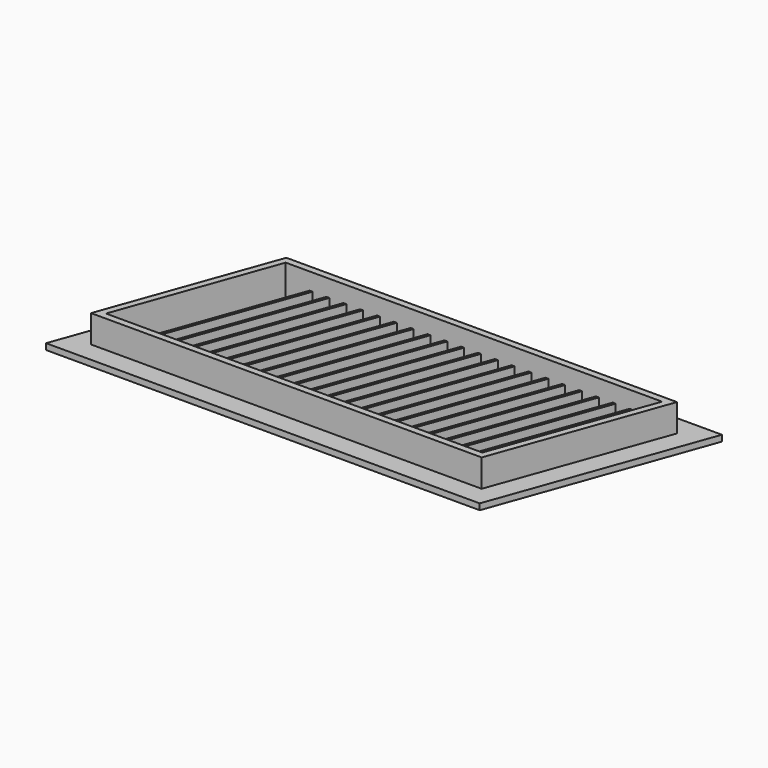
from build123d import *

# Parameters (mm, degrees)
F1_DEPTH      = 1.8
F2_DEPTH      = 5
F3_DEPTH      = 10
F4_T4_DEPTH   = 59.1767472924
F4_T10_DEPTH  = 59.1767472924
F4_T16_DEPTH  = 59.1767472924
F4_T22_DEPTH  = 59.1767472924
F4_T28_DEPTH  = 59.1767472924
F4_T34_DEPTH  = 59.1767472924
F4_T40_DEPTH  = 59.1767472924
F4_T46_DEPTH  = 59.1767472924
F4_T52_DEPTH  = 59.1767472924
F4_T58_DEPTH  = 59.1767472924
F4_T64_DEPTH  = 59.1767472924
F4_T70_DEPTH  = 59.1767472924
F4_T76_DEPTH  = 59.1767472924
F4_T82_DEPTH  = 59.1767472924
F4_T88_DEPTH  = 59.1767472924
F4_T94_DEPTH  = 59.1767472924
F4_T100_DEPTH = 59.1767472924
F4_T106_DEPTH = 59.1767472924
F4_T112_DEPTH = 59.1767472924
F4_T118_DEPTH = 59.1767472924
F4_T124_DEPTH = 59.1767472924
F4_T130_DEPTH = 59.1767472924
F4_T136_DEPTH = 59.1767472924
F4_T142_DEPTH = 59.1767472924
F4_T148_DEPTH = 59.1767472924
F4_T154_DEPTH = 59.1767472924
F4_T160_DEPTH = 59.1767472924
F4_T166_DEPTH = 59.1767472924
F4_T172_DEPTH = 59.1767472924
F4_T178_DEPTH = 59.1767472924
F4_T184_DEPTH = 59.1767472924
F4_T190_DEPTH = 59.1767472924
F4_T196_DEPTH = 59.1767472924
F4_T202_DEPTH = 59.1767472924
F4_T208_DEPTH = 59.1767472924
F4_T214_DEPTH = 59.1767472924
F4_T220_DEPTH = 59.1767472924
F4_T226_DEPTH = 59.1767472924
F4_T232_DEPTH = 59.1767472924
F4_T238_DEPTH = 59.1767472924
F4_T244_DEPTH = 59.1767472924
F4_T250_DEPTH = 59.1767472924
F4_T256_DEPTH = 59.1767472924


# Not quite as in the source:
# - a fillet or chamfer that OpenCascade refuses, or shapes differently, is made with other operations: its cross-section is extruded or revolved along the edge and cut away or added
# - a feature names something its author has since deleted; it is built from what else it names


with BuildPart() as f1:
    # F0 (on Top) → F1 (new body)
    with BuildSketch(Plane.XY):
        Polygon((4.2169585227, -6), (26.5369585227, 56), (-102.2169585227, 56), (-124.5369585227, -6), align=None)
        Polygon((-98, 0), (-116, 0), (-98, 50), (18, 50), (0, 0), align=None, mode=Mode.SUBTRACT)
    extrude(amount=F1_DEPTH)

    # F0 (on Top) → F2 (join)
    with BuildSketch(Plane.XY):
        Polygon((-98, 50), (-116, 0), (-98, 0), (0, 0), (18, 50), align=None)
        Polygon((13.4056528409, 48), (15.1543471591, 48), (-1.4056528409, 2), (-3.1543471591, 2), (-5.1543471591, 2), (-8.1543471591, 2), (-10.1543471591, 2), (-13.1543471591, 2), (-15.1543471591, 2), (-18.1543471591, 2), (-20.1543471591, 2), (-23.1543471591, 2), (-25.1543471591, 2), (-28.1543471591, 2), (-30.1543471591, 2), (-33.1543471591, 2), (-35.1543471591, 2), (-38.1543471591, 2), (-40.1543471591, 2), (-43.1543471591, 2), (-45.1543471591, 2), (-48.1543471591, 2), (-50.1543471591, 2), (-53.1543471591, 2), (-55.1543471591, 2), (-58.1543471591, 2), (-60.1543471591, 2), (-63.1543471591, 2), (-65.1543471591, 2), (-68.1543471591, 2), (-70.1543471591, 2), (-73.1543471591, 2), (-75.1543471591, 2), (-78.1543471591, 2), (-80.1543471591, 2), (-83.1543471591, 2), (-85.1543471591, 2), (-88.1543471591, 2), (-90.1543471591, 2), (-93.1543471591, 2), (-95.1543471591, 2), (-98.1543471591, 2), (-100.1543471591, 2), (-103.1543471591, 2), (-105.1543471591, 2), (-108.1543471591, 2), (-113.1543471591, 2), (-96.5943471591, 48), (-91.5943471591, 48), (-88.5943471591, 48), (-86.5943471591, 48), (-83.5943471591, 48), (-81.5943471591, 48), (-78.5943471591, 48), (-76.5943471591, 48), (-73.5943471591, 48), (-71.5943471591, 48), (-68.5943471591, 48), (-66.5943471591, 48), (-63.5943471591, 48), (-61.5943471591, 48), (-58.5943471591, 48), (-56.5943471591, 48), (-53.5943471591, 48), (-51.5943471591, 48), (-48.5943471591, 48), (-46.5943471591, 48), (-43.5943471591, 48), (-41.5943471591, 48), (-38.5943471591, 48), (-36.5943471591, 48), (-33.5943471591, 48), (-31.5943471591, 48), (-28.5943471591, 48), (-26.5943471591, 48), (-23.5943471591, 48), (-21.5943471591, 48), (-18.5943471591, 48), (-16.5943471591, 48), (-13.5943471591, 48), (-11.5943471591, 48), (-8.5943471591, 48), (-6.5943471591, 48), (-3.5943471591, 48), (-1.5943471591, 48), (1.4056528409, 48), (3.4056528409, 48), (6.4056528409, 48), (8.4056528409, 48), (11.4056528409, 48), align=None, mode=Mode.SUBTRACT)
        Polygon((-105.1543471591, 2), (-88.5943471591, 48), (-91.5943471591, 48), (-108.1543471591, 2), align=None)
        Polygon((-100.1543471591, 2), (-83.5943471591, 48), (-86.5943471591, 48), (-103.1543471591, 2), align=None)
        Polygon((-95.1543471591, 2), (-78.5943471591, 48), (-81.5943471591, 48), (-98.1543471591, 2), align=None)
        Polygon((-90.1543471591, 2), (-73.5943471591, 48), (-76.5943471591, 48), (-93.1543471591, 2), align=None)
        Polygon((-85.1543471591, 2), (-68.5943471591, 48), (-71.5943471591, 48), (-88.1543471591, 2), align=None)
        Polygon((-80.1543471591, 2), (-63.5943471591, 48), (-66.5943471591, 48), (-83.1543471591, 2), align=None)
        Polygon((-75.1543471591, 2), (-58.5943471591, 48), (-61.5943471591, 48), (-78.1543471591, 2), align=None)
        Polygon((-70.1543471591, 2), (-53.5943471591, 48), (-56.5943471591, 48), (-73.1543471591, 2), align=None)
        Polygon((-65.1543471591, 2), (-48.5943471591, 48), (-51.5943471591, 48), (-68.1543471591, 2), align=None)
        Polygon((-60.1543471591, 2), (-43.5943471591, 48), (-46.5943471591, 48), (-63.1543471591, 2), align=None)
        Polygon((-55.1543471591, 2), (-38.5943471591, 48), (-41.5943471591, 48), (-58.1543471591, 2), align=None)
        Polygon((-50.1543471591, 2), (-33.5943471591, 48), (-36.5943471591, 48), (-53.1543471591, 2), align=None)
        Polygon((-45.1543471591, 2), (-28.5943471591, 48), (-31.5943471591, 48), (-48.1543471591, 2), align=None)
        Polygon((-40.1543471591, 2), (-23.5943471591, 48), (-26.5943471591, 48), (-43.1543471591, 2), align=None)
        Polygon((-35.1543471591, 2), (-18.5943471591, 48), (-21.5943471591, 48), (-38.1543471591, 2), align=None)
        Polygon((-30.1543471591, 2), (-13.5943471591, 48), (-16.5943471591, 48), (-33.1543471591, 2), align=None)
        Polygon((-25.1543471591, 2), (-8.5943471591, 48), (-11.5943471591, 48), (-28.1543471591, 2), align=None)
        Polygon((-20.1543471591, 2), (-3.5943471591, 48), (-6.5943471591, 48), (-23.1543471591, 2), align=None)
        Polygon((-15.1543471591, 2), (1.4056528409, 48), (-1.5943471591, 48), (-18.1543471591, 2), align=None)
        Polygon((-10.1543471591, 2), (6.4056528409, 48), (3.4056528409, 48), (-13.1543471591, 2), align=None)
        Polygon((-5.1543471591, 2), (11.4056528409, 48), (8.4056528409, 48), (-8.1543471591, 2), align=None)
        Polygon((-1.4056528409, 2), (15.1543471591, 48), (13.4056528409, 48), (-3.1543471591, 2), align=None)
    extrude(amount=F2_DEPTH)

    # F0 (on Top) → F3 (join)
    with BuildSketch(Plane.XY):
        Polygon((-98, 50), (-116, 0), (-98, 0), (0, 0), (18, 50), align=None)
        Polygon((13.4056528409, 48), (15.1543471591, 48), (-1.4056528409, 2), (-3.1543471591, 2), (-5.1543471591, 2), (-8.1543471591, 2), (-10.1543471591, 2), (-13.1543471591, 2), (-15.1543471591, 2), (-18.1543471591, 2), (-20.1543471591, 2), (-23.1543471591, 2), (-25.1543471591, 2), (-28.1543471591, 2), (-30.1543471591, 2), (-33.1543471591, 2), (-35.1543471591, 2), (-38.1543471591, 2), (-40.1543471591, 2), (-43.1543471591, 2), (-45.1543471591, 2), (-48.1543471591, 2), (-50.1543471591, 2), (-53.1543471591, 2), (-55.1543471591, 2), (-58.1543471591, 2), (-60.1543471591, 2), (-63.1543471591, 2), (-65.1543471591, 2), (-68.1543471591, 2), (-70.1543471591, 2), (-73.1543471591, 2), (-75.1543471591, 2), (-78.1543471591, 2), (-80.1543471591, 2), (-83.1543471591, 2), (-85.1543471591, 2), (-88.1543471591, 2), (-90.1543471591, 2), (-93.1543471591, 2), (-95.1543471591, 2), (-98.1543471591, 2), (-100.1543471591, 2), (-103.1543471591, 2), (-105.1543471591, 2), (-108.1543471591, 2), (-113.1543471591, 2), (-96.5943471591, 48), (-91.5943471591, 48), (-88.5943471591, 48), (-86.5943471591, 48), (-83.5943471591, 48), (-81.5943471591, 48), (-78.5943471591, 48), (-76.5943471591, 48), (-73.5943471591, 48), (-71.5943471591, 48), (-68.5943471591, 48), (-66.5943471591, 48), (-63.5943471591, 48), (-61.5943471591, 48), (-58.5943471591, 48), (-56.5943471591, 48), (-53.5943471591, 48), (-51.5943471591, 48), (-48.5943471591, 48), (-46.5943471591, 48), (-43.5943471591, 48), (-41.5943471591, 48), (-38.5943471591, 48), (-36.5943471591, 48), (-33.5943471591, 48), (-31.5943471591, 48), (-28.5943471591, 48), (-26.5943471591, 48), (-23.5943471591, 48), (-21.5943471591, 48), (-18.5943471591, 48), (-16.5943471591, 48), (-13.5943471591, 48), (-11.5943471591, 48), (-8.5943471591, 48), (-6.5943471591, 48), (-3.5943471591, 48), (-1.5943471591, 48), (1.4056528409, 48), (3.4056528409, 48), (6.4056528409, 48), (8.4056528409, 48), (11.4056528409, 48), align=None, mode=Mode.SUBTRACT)
    extrude(amount=F3_DEPTH)

    # F4: chamfer of 2 on 43 edges, made by hand


with BuildPart() as f4_tool2:
    # F4_s3 → F4_t4 (new body)
    with BuildSketch(Plane(origin=(-8.0063254971, -22.2397930476, 0), x_dir=(0, 0, 1), z_dir=(0.3387194683, 0.9408874119, 0))):
        Polygon((2, -57.2759069477), (0, -59.2759069477), (0, -57.2759069477), align=None)
    extrude(amount=F4_T4_DEPTH)

    split(bisect_by=Plane.XZ.offset(-2), keep=Keep.BOTTOM)

    split(bisect_by=Plane.XZ.offset(-48), keep=Keep.TOP)


with BuildPart() as f1_1:
    add(f1.part)

    # F4_t1: cut F4_tool2
    add(f4_tool2.part, mode=Mode.SUBTRACT)


with BuildPart() as f4_tool8:
    # F4_s9 → F4_t10 (new body)
    with BuildSketch(Plane(origin=(-8.5799798881, -23.8332774668, 0), x_dir=(0, 0, 1), z_dir=(0.3387194683, 0.9408874119, 0))):
        Polygon((2, -61.9803440071), (0, -63.9803440071), (0, -61.9803440071), align=None)
    extrude(amount=F4_T10_DEPTH)

    split(bisect_by=Plane.XZ.offset(-2), keep=Keep.BOTTOM)

    split(bisect_by=Plane.XZ.offset(-48), keep=Keep.TOP)


with BuildPart() as f1_2:
    add(f1_1.part)

    # F4_t7: cut F4_tool8
    add(f4_tool8.part, mode=Mode.SUBTRACT)


with BuildPart() as f4_tool14:
    # F4_s15 → F4_t16 (new body)
    with BuildSketch(Plane(origin=(-9.153634279, -25.4267618861, 0), x_dir=(0, 0, 1), z_dir=(0.3387194683, 0.9408874119, 0))):
        Polygon((2, -66.6847810664), (0, -68.6847810664), (0, -66.6847810664), align=None)
    extrude(amount=F4_T16_DEPTH)

    split(bisect_by=Plane.XZ.offset(-2), keep=Keep.BOTTOM)

    split(bisect_by=Plane.XZ.offset(-48), keep=Keep.TOP)


with BuildPart() as f1_3:
    add(f1_2.part)

    # F4_t13: cut F4_tool14
    add(f4_tool14.part, mode=Mode.SUBTRACT)


with BuildPart() as f4_tool20:
    # F4_s21 → F4_t22 (new body)
    with BuildSketch(Plane(origin=(-9.7272886699, -27.0202463054, 0), x_dir=(0, 0, 1), z_dir=(0.3387194683, 0.9408874119, 0))):
        Polygon((2, -71.3892181258), (0, -73.3892181258), (0, -71.3892181258), align=None)
    extrude(amount=F4_T22_DEPTH)

    split(bisect_by=Plane.XZ.offset(-2), keep=Keep.BOTTOM)

    split(bisect_by=Plane.XZ.offset(-48), keep=Keep.TOP)


with BuildPart() as f1_4:
    add(f1_3.part)

    # F4_t19: cut F4_tool20
    add(f4_tool20.part, mode=Mode.SUBTRACT)


with BuildPart() as f4_tool26:
    # F4_s27 → F4_t28 (new body)
    with BuildSketch(Plane(origin=(-10.3009430609, -28.6137307246, 0), x_dir=(0, 0, 1), z_dir=(0.3387194683, 0.9408874119, 0))):
        Polygon((2, -76.0936551851), (0, -78.0936551851), (0, -76.0936551851), align=None)
    extrude(amount=F4_T28_DEPTH)

    split(bisect_by=Plane.XZ.offset(-2), keep=Keep.BOTTOM)

    split(bisect_by=Plane.XZ.offset(-48), keep=Keep.TOP)


with BuildPart() as f1_5:
    add(f1_4.part)

    # F4_t25: cut F4_tool26
    add(f4_tool26.part, mode=Mode.SUBTRACT)


with BuildPart() as f4_tool32:
    # F4_s33 → F4_t34 (new body)
    with BuildSketch(Plane(origin=(-10.8745974518, -30.2072151439, 0), x_dir=(0, 0, 1), z_dir=(0.3387194683, 0.9408874119, 0))):
        Polygon((2, -80.7980922444), (0, -82.7980922444), (0, -80.7980922444), align=None)
    extrude(amount=F4_T34_DEPTH)

    split(bisect_by=Plane.XZ.offset(-2), keep=Keep.BOTTOM)

    split(bisect_by=Plane.XZ.offset(-48), keep=Keep.TOP)


with BuildPart() as f1_6:
    add(f1_5.part)

    # F4_t31: cut F4_tool32
    add(f4_tool32.part, mode=Mode.SUBTRACT)


with BuildPart() as f4_tool38:
    # F4_s39 → F4_t40 (new body)
    with BuildSketch(Plane(origin=(-11.4482518427, -31.8006995631, 0), x_dir=(0, 0, 1), z_dir=(0.3387194683, 0.9408874119, 0))):
        Polygon((2, -85.5025293038), (0, -87.5025293038), (0, -85.5025293038), align=None)
    extrude(amount=F4_T40_DEPTH)

    split(bisect_by=Plane.XZ.offset(-2), keep=Keep.BOTTOM)

    split(bisect_by=Plane.XZ.offset(-48), keep=Keep.TOP)


with BuildPart() as f1_7:
    add(f1_6.part)

    # F4_t37: cut F4_tool38
    add(f4_tool38.part, mode=Mode.SUBTRACT)


with BuildPart() as f4_tool44:
    # F4_s45 → F4_t46 (new body)
    with BuildSketch(Plane(origin=(-12.0219062337, -33.3941839824, 0), x_dir=(0, 0, 1), z_dir=(0.3387194683, 0.9408874119, 0))):
        Polygon((2, -90.2069663631), (0, -92.2069663631), (0, -90.2069663631), align=None)
    extrude(amount=F4_T46_DEPTH)

    split(bisect_by=Plane.XZ.offset(-2), keep=Keep.BOTTOM)

    split(bisect_by=Plane.XZ.offset(-48), keep=Keep.TOP)


with BuildPart() as f1_8:
    add(f1_7.part)

    # F4_t43: cut F4_tool44
    add(f4_tool44.part, mode=Mode.SUBTRACT)


with BuildPart() as f4_tool50:
    # F4_s51 → F4_t52 (new body)
    with BuildSketch(Plane(origin=(-12.5955606246, -34.9876684017, 0), x_dir=(0, 0, 1), z_dir=(0.3387194683, 0.9408874119, 0))):
        Polygon((2, -94.9114034225), (0, -96.9114034225), (0, -94.9114034225), align=None)
    extrude(amount=F4_T52_DEPTH)

    split(bisect_by=Plane.XZ.offset(-2), keep=Keep.BOTTOM)

    split(bisect_by=Plane.XZ.offset(-48), keep=Keep.TOP)


with BuildPart() as f1_9:
    add(f1_8.part)

    # F4_t49: cut F4_tool50
    add(f4_tool50.part, mode=Mode.SUBTRACT)


with BuildPart() as f4_tool56:
    # F4_s57 → F4_t58 (new body)
    with BuildSketch(Plane(origin=(-13.1692150155, -36.5811528209, 0), x_dir=(0, 0, 1), z_dir=(0.3387194683, 0.9408874119, 0))):
        Polygon((2, -99.6158404818), (0, -101.6158404818), (0, -99.6158404818), align=None)
    extrude(amount=F4_T58_DEPTH)

    split(bisect_by=Plane.XZ.offset(-2), keep=Keep.BOTTOM)

    split(bisect_by=Plane.XZ.offset(-48), keep=Keep.TOP)


with BuildPart() as f1_10:
    add(f1_9.part)

    # F4_t55: cut F4_tool56
    add(f4_tool56.part, mode=Mode.SUBTRACT)


with BuildPart() as f4_tool62:
    # F4_s63 → F4_t64 (new body)
    with BuildSketch(Plane(origin=(11.6937982453, 32.4827729037, 0), x_dir=(0, 0, 1), z_dir=(-0.3387194683, -0.9408874119, 0))):
        Polygon((5, 58.0985691833), (3, 60.0985691833), (5, 60.0985691833), align=None)
    extrude(amount=F4_T64_DEPTH)

    split(bisect_by=Plane.XZ.offset(-2), keep=Keep.BOTTOM)

    split(bisect_by=Plane.XZ.offset(-48), keep=Keep.TOP)


with BuildPart() as f1_11:
    add(f1_10.part)

    # F4_t61: cut F4_tool62
    add(f4_tool62.part, mode=Mode.SUBTRACT)


with BuildPart() as f4_tool68:
    # F4_s69 → F4_t70 (new body)
    with BuildSketch(Plane(origin=(11.1201438544, 30.8892884844, 0), x_dir=(0, 0, 1), z_dir=(-0.3387194683, -0.9408874119, 0))):
        Polygon((5, 62.8030062427), (3, 64.8030062427), (5, 64.8030062427), align=None)
    extrude(amount=F4_T70_DEPTH)

    split(bisect_by=Plane.XZ.offset(-2), keep=Keep.BOTTOM)

    split(bisect_by=Plane.XZ.offset(-48), keep=Keep.TOP)


with BuildPart() as f1_12:
    add(f1_11.part)

    # F4_t67: cut F4_tool68
    add(f4_tool68.part, mode=Mode.SUBTRACT)


with BuildPart() as f4_tool74:
    # F4_s75 → F4_t76 (new body)
    with BuildSketch(Plane(origin=(10.5464894634, 29.2958040651, 0), x_dir=(0, 0, 1), z_dir=(-0.3387194683, -0.9408874119, 0))):
        Polygon((5, 67.507443302), (3, 69.507443302), (5, 69.507443302), align=None)
    extrude(amount=F4_T76_DEPTH)

    split(bisect_by=Plane.XZ.offset(-2), keep=Keep.BOTTOM)

    split(bisect_by=Plane.XZ.offset(-48), keep=Keep.TOP)


with BuildPart() as f1_13:
    add(f1_12.part)

    # F4_t73: cut F4_tool74
    add(f4_tool74.part, mode=Mode.SUBTRACT)


with BuildPart() as f4_tool80:
    # F4_s81 → F4_t82 (new body)
    with BuildSketch(Plane(origin=(9.9728350725, 27.7023196459, 0), x_dir=(0, 0, 1), z_dir=(-0.3387194683, -0.9408874119, 0))):
        Polygon((5, 72.2118803614), (3, 74.2118803614), (5, 74.2118803614), align=None)
    extrude(amount=F4_T82_DEPTH)

    split(bisect_by=Plane.XZ.offset(-2), keep=Keep.BOTTOM)

    split(bisect_by=Plane.XZ.offset(-48), keep=Keep.TOP)


with BuildPart() as f1_14:
    add(f1_13.part)

    # F4_t79: cut F4_tool80
    add(f4_tool80.part, mode=Mode.SUBTRACT)


with BuildPart() as f4_tool86:
    # F4_s87 → F4_t88 (new body)
    with BuildSketch(Plane(origin=(9.3991806816, 26.1088352266, 0), x_dir=(0, 0, 1), z_dir=(-0.3387194683, -0.9408874119, 0))):
        Polygon((5, 76.9163174207), (3, 78.9163174207), (5, 78.9163174207), align=None)
    extrude(amount=F4_T88_DEPTH)

    split(bisect_by=Plane.XZ.offset(-2), keep=Keep.BOTTOM)

    split(bisect_by=Plane.XZ.offset(-48), keep=Keep.TOP)


with BuildPart() as f1_15:
    add(f1_14.part)

    # F4_t85: cut F4_tool86
    add(f4_tool86.part, mode=Mode.SUBTRACT)


with BuildPart() as f4_tool92:
    # F4_s93 → F4_t94 (new body)
    with BuildSketch(Plane(origin=(8.8255262906, 24.5153508073, 0), x_dir=(0, 0, 1), z_dir=(-0.3387194683, -0.9408874119, 0))):
        Polygon((5, 81.6207544801), (3, 83.6207544801), (5, 83.6207544801), align=None)
    extrude(amount=F4_T94_DEPTH)

    split(bisect_by=Plane.XZ.offset(-2), keep=Keep.BOTTOM)

    split(bisect_by=Plane.XZ.offset(-48), keep=Keep.TOP)


with BuildPart() as f1_16:
    add(f1_15.part)

    # F4_t91: cut F4_tool92
    add(f4_tool92.part, mode=Mode.SUBTRACT)


with BuildPart() as f4_tool98:
    # F4_s99 → F4_t100 (new body)
    with BuildSketch(Plane(origin=(8.2518718997, 22.9218663881, 0), x_dir=(0, 0, 1), z_dir=(-0.3387194683, -0.9408874119, 0))):
        Polygon((5, 86.3251915394), (3, 88.3251915394), (5, 88.3251915394), align=None)
    extrude(amount=F4_T100_DEPTH)

    split(bisect_by=Plane.XZ.offset(-2), keep=Keep.BOTTOM)

    split(bisect_by=Plane.XZ.offset(-48), keep=Keep.TOP)


with BuildPart() as f1_17:
    add(f1_16.part)

    # F4_t97: cut F4_tool98
    add(f4_tool98.part, mode=Mode.SUBTRACT)


with BuildPart() as f4_tool104:
    # F4_s105 → F4_t106 (new body)
    with BuildSketch(Plane(origin=(7.6782175088, 21.3283819688, 0), x_dir=(0, 0, 1), z_dir=(-0.3387194683, -0.9408874119, 0))):
        Polygon((5, 91.0296285987), (3, 93.0296285987), (5, 93.0296285987), align=None)
    extrude(amount=F4_T106_DEPTH)

    split(bisect_by=Plane.XZ.offset(-2), keep=Keep.BOTTOM)

    split(bisect_by=Plane.XZ.offset(-48), keep=Keep.TOP)


with BuildPart() as f1_18:
    add(f1_17.part)

    # F4_t103: cut F4_tool104
    add(f4_tool104.part, mode=Mode.SUBTRACT)


with BuildPart() as f4_tool110:
    # F4_s111 → F4_t112 (new body)
    with BuildSketch(Plane(origin=(7.1045631178, 19.7348975495, 0), x_dir=(0, 0, 1), z_dir=(-0.3387194683, -0.9408874119, 0))):
        Polygon((5, 95.7340656581), (3, 97.7340656581), (5, 97.7340656581), align=None)
    extrude(amount=F4_T112_DEPTH)

    split(bisect_by=Plane.XZ.offset(-2), keep=Keep.BOTTOM)

    split(bisect_by=Plane.XZ.offset(-48), keep=Keep.TOP)


with BuildPart() as f1_19:
    add(f1_18.part)

    # F4_t109: cut F4_tool110
    add(f4_tool110.part, mode=Mode.SUBTRACT)


with BuildPart() as f4_tool116:
    # F4_s117 → F4_t118 (new body)
    with BuildSketch(Plane(origin=(6.5309087269, 18.1414131303, 0), x_dir=(0, 0, 1), z_dir=(-0.3387194683, -0.9408874119, 0))):
        Polygon((5, 100.4385027174), (3, 102.4385027174), (5, 102.4385027174), align=None)
    extrude(amount=F4_T118_DEPTH)

    split(bisect_by=Plane.XZ.offset(-2), keep=Keep.BOTTOM)

    split(bisect_by=Plane.XZ.offset(-48), keep=Keep.TOP)


with BuildPart() as f1_20:
    add(f1_19.part)

    # F4_t115: cut F4_tool116
    add(f4_tool116.part, mode=Mode.SUBTRACT)


with BuildPart() as f4_tool122:
    # F4_s123 → F4_t124 (new body)
    with BuildSketch(Plane(origin=(-7.4326711062, -20.6463086283, 0), x_dir=(0, 0, 1), z_dir=(0.3387194683, 0.9408874119, 0))):
        Polygon((2, -52.5714698884), (0, -54.5714698884), (0, -52.5714698884), align=None)
    extrude(amount=F4_T124_DEPTH)

    split(bisect_by=Plane.XZ.offset(-2), keep=Keep.BOTTOM)

    split(bisect_by=Plane.XZ.offset(-48), keep=Keep.TOP)


with BuildPart() as f1_21:
    add(f1_20.part)

    # F4_t121: cut F4_tool122
    add(f4_tool122.part, mode=Mode.SUBTRACT)


with BuildPart() as f4_tool128:
    # F4_s129 → F4_t130 (new body)
    with BuildSketch(Plane(origin=(-6.8590167153, -19.052824209, 0), x_dir=(0, 0, 1), z_dir=(0.3387194683, 0.9408874119, 0))):
        Polygon((2, -47.867032829), (0, -49.867032829), (0, -47.867032829), align=None)
    extrude(amount=F4_T130_DEPTH)

    split(bisect_by=Plane.XZ.offset(-2), keep=Keep.BOTTOM)

    split(bisect_by=Plane.XZ.offset(-48), keep=Keep.TOP)


with BuildPart() as f1_22:
    add(f1_21.part)

    # F4_t127: cut F4_tool128
    add(f4_tool128.part, mode=Mode.SUBTRACT)


with BuildPart() as f4_tool134:
    # F4_s135 → F4_t136 (new body)
    with BuildSketch(Plane(origin=(-6.2853623243, -17.4593397898, 0), x_dir=(0, 0, 1), z_dir=(0.3387194683, 0.9408874119, 0))):
        Polygon((2, -43.1625957697), (0, -45.1625957697), (0, -43.1625957697), align=None)
    extrude(amount=F4_T136_DEPTH)

    split(bisect_by=Plane.XZ.offset(-2), keep=Keep.BOTTOM)

    split(bisect_by=Plane.XZ.offset(-48), keep=Keep.TOP)


with BuildPart() as f1_23:
    add(f1_22.part)

    # F4_t133: cut F4_tool134
    add(f4_tool134.part, mode=Mode.SUBTRACT)


with BuildPart() as f4_tool140:
    # F4_s141 → F4_t142 (new body)
    with BuildSketch(Plane(origin=(-5.7117079334, -15.8658553705, 0), x_dir=(0, 0, 1), z_dir=(0.3387194683, 0.9408874119, 0))):
        Polygon((2, -38.4581587104), (0, -40.4581587104), (0, -38.4581587104), align=None)
    extrude(amount=F4_T142_DEPTH)

    split(bisect_by=Plane.XZ.offset(-2), keep=Keep.BOTTOM)

    split(bisect_by=Plane.XZ.offset(-48), keep=Keep.TOP)


with BuildPart() as f1_24:
    add(f1_23.part)

    # F4_t139: cut F4_tool140
    add(f4_tool140.part, mode=Mode.SUBTRACT)


with BuildPart() as f4_tool146:
    # F4_s147 → F4_t148 (new body)
    with BuildSketch(Plane(origin=(-5.1380535424, -14.2723709512, 0), x_dir=(0, 0, 1), z_dir=(0.3387194683, 0.9408874119, 0))):
        Polygon((2, -33.753721651), (0, -35.753721651), (0, -33.753721651), align=None)
    extrude(amount=F4_T148_DEPTH)

    split(bisect_by=Plane.XZ.offset(-2), keep=Keep.BOTTOM)

    split(bisect_by=Plane.XZ.offset(-48), keep=Keep.TOP)


with BuildPart() as f1_25:
    add(f1_24.part)

    # F4_t145: cut F4_tool146
    add(f4_tool146.part, mode=Mode.SUBTRACT)


with BuildPart() as f4_tool152:
    # F4_s153 → F4_t154 (new body)
    with BuildSketch(Plane(origin=(-4.5643991515, -12.678886532, 0), x_dir=(0, 0, 1), z_dir=(0.3387194683, 0.9408874119, 0))):
        Polygon((2, -29.0492845917), (0, -31.0492845917), (0, -29.0492845917), align=None)
    extrude(amount=F4_T154_DEPTH)

    split(bisect_by=Plane.XZ.offset(-2), keep=Keep.BOTTOM)

    split(bisect_by=Plane.XZ.offset(-48), keep=Keep.TOP)


with BuildPart() as f1_26:
    add(f1_25.part)

    # F4_t151: cut F4_tool152
    add(f4_tool152.part, mode=Mode.SUBTRACT)


with BuildPart() as f4_tool158:
    # F4_s159 → F4_t160 (new body)
    with BuildSketch(Plane(origin=(-3.9907447606, -11.0854021127, 0), x_dir=(0, 0, 1), z_dir=(0.3387194683, 0.9408874119, 0))):
        Polygon((2, -24.3448475323), (0, -26.3448475323), (0, -24.3448475323), align=None)
    extrude(amount=F4_T160_DEPTH)

    split(bisect_by=Plane.XZ.offset(-2), keep=Keep.BOTTOM)

    split(bisect_by=Plane.XZ.offset(-48), keep=Keep.TOP)


with BuildPart() as f1_27:
    add(f1_26.part)

    # F4_t157: cut F4_tool158
    add(f4_tool158.part, mode=Mode.SUBTRACT)


with BuildPart() as f4_tool164:
    # F4_s165 → F4_t166 (new body)
    with BuildSketch(Plane(origin=(-3.4170903696, -9.4919176935, 0), x_dir=(0, 0, 1), z_dir=(0.3387194683, 0.9408874119, 0))):
        Polygon((2, -19.640410473), (0, -21.640410473), (0, -19.640410473), align=None)
    extrude(amount=F4_T166_DEPTH)

    split(bisect_by=Plane.XZ.offset(-2), keep=Keep.BOTTOM)

    split(bisect_by=Plane.XZ.offset(-48), keep=Keep.TOP)


with BuildPart() as f1_28:
    add(f1_27.part)

    # F4_t163: cut F4_tool164
    add(f4_tool164.part, mode=Mode.SUBTRACT)


with BuildPart() as f4_tool170:
    # F4_s171 → F4_t172 (new body)
    with BuildSketch(Plane(origin=(-2.8434359787, -7.8984332742, 0), x_dir=(0, 0, 1), z_dir=(0.3387194683, 0.9408874119, 0))):
        Polygon((2, -14.9359734136), (0, -16.9359734136), (0, -14.9359734136), align=None)
    extrude(amount=F4_T172_DEPTH)

    split(bisect_by=Plane.XZ.offset(-2), keep=Keep.BOTTOM)

    split(bisect_by=Plane.XZ.offset(-48), keep=Keep.TOP)


with BuildPart() as f1_29:
    add(f1_28.part)

    # F4_t169: cut F4_tool170
    add(f4_tool170.part, mode=Mode.SUBTRACT)


with BuildPart() as f4_tool176:
    # F4_s177 → F4_t178 (new body)
    with BuildSketch(Plane(origin=(-2.2697815878, -6.3049488549, 0), x_dir=(0, 0, 1), z_dir=(0.3387194683, 0.9408874119, 0))):
        Polygon((2, -10.2315363543), (0, -12.2315363543), (0, -10.2315363543), align=None)
    extrude(amount=F4_T178_DEPTH)

    split(bisect_by=Plane.XZ.offset(-2), keep=Keep.BOTTOM)

    split(bisect_by=Plane.XZ.offset(-48), keep=Keep.TOP)


with BuildPart() as f1_30:
    add(f1_29.part)

    # F4_t175: cut F4_tool176
    add(f4_tool176.part, mode=Mode.SUBTRACT)


with BuildPart() as f4_tool182:
    # F4_s183 → F4_t184 (new body)
    with BuildSketch(Plane(origin=(-1.6961271968, -4.7114644357, 0), x_dir=(0, 0, 1), z_dir=(0.3387194683, 0.9408874119, 0))):
        Polygon((2, -5.527099295), (0, -7.527099295), (0, -5.527099295), align=None)
    extrude(amount=F4_T184_DEPTH)

    split(bisect_by=Plane.XZ.offset(-2), keep=Keep.BOTTOM)

    split(bisect_by=Plane.XZ.offset(-48), keep=Keep.TOP)


with BuildPart() as f1_31:
    add(f1_30.part)

    # F4_t181: cut F4_tool182
    add(f4_tool182.part, mode=Mode.SUBTRACT)


with BuildPart() as f4_tool188:
    # F4_s189 → F4_t190 (new body)
    with BuildSketch(Plane(origin=(12.2674526363, 34.0762573229, 0), x_dir=(0, 0, 1), z_dir=(-0.3387194683, -0.9408874119, 0))):
        Polygon((5, 53.394132124), (3, 55.394132124), (5, 55.394132124), align=None)
    extrude(amount=F4_T190_DEPTH)

    split(bisect_by=Plane.XZ.offset(-2), keep=Keep.BOTTOM)

    split(bisect_by=Plane.XZ.offset(-48), keep=Keep.TOP)


with BuildPart() as f1_32:
    add(f1_31.part)

    # F4_t187: cut F4_tool188
    add(f4_tool188.part, mode=Mode.SUBTRACT)


with BuildPart() as f4_tool194:
    # F4_s195 → F4_t196 (new body)
    with BuildSketch(Plane(origin=(12.8411070272, 35.6697417422, 0), x_dir=(0, 0, 1), z_dir=(-0.3387194683, -0.9408874119, 0))):
        Polygon((5, 48.6896950646), (3, 50.6896950646), (5, 50.6896950646), align=None)
    extrude(amount=F4_T196_DEPTH)

    split(bisect_by=Plane.XZ.offset(-2), keep=Keep.BOTTOM)

    split(bisect_by=Plane.XZ.offset(-48), keep=Keep.TOP)


with BuildPart() as f1_33:
    add(f1_32.part)

    # F4_t193: cut F4_tool194
    add(f4_tool194.part, mode=Mode.SUBTRACT)


with BuildPart() as f4_tool200:
    # F4_s201 → F4_t202 (new body)
    with BuildSketch(Plane(origin=(13.4147614181, 37.2632261614, 0), x_dir=(0, 0, 1), z_dir=(-0.3387194683, -0.9408874119, 0))):
        Polygon((5, 43.9852580053), (3, 45.9852580053), (5, 45.9852580053), align=None)
    extrude(amount=F4_T202_DEPTH)

    split(bisect_by=Plane.XZ.offset(-2), keep=Keep.BOTTOM)

    split(bisect_by=Plane.XZ.offset(-48), keep=Keep.TOP)


with BuildPart() as f1_34:
    add(f1_33.part)

    # F4_t199: cut F4_tool200
    add(f4_tool200.part, mode=Mode.SUBTRACT)


with BuildPart() as f4_tool206:
    # F4_s207 → F4_t208 (new body)
    with BuildSketch(Plane(origin=(13.9884158091, 38.8567105807, 0), x_dir=(0, 0, 1), z_dir=(-0.3387194683, -0.9408874119, 0))):
        Polygon((5, 39.280820946), (3, 41.280820946), (5, 41.280820946), align=None)
    extrude(amount=F4_T208_DEPTH)

    split(bisect_by=Plane.XZ.offset(-2), keep=Keep.BOTTOM)

    split(bisect_by=Plane.XZ.offset(-48), keep=Keep.TOP)


with BuildPart() as f1_35:
    add(f1_34.part)

    # F4_t205: cut F4_tool206
    add(f4_tool206.part, mode=Mode.SUBTRACT)


with BuildPart() as f4_tool212:
    # F4_s213 → F4_t214 (new body)
    with BuildSketch(Plane(origin=(14.5620702, 40.450195, 0), x_dir=(0, 0, 1), z_dir=(-0.3387194683, -0.9408874119, 0))):
        Polygon((5, 34.5763838866), (3, 36.5763838866), (5, 36.5763838866), align=None)
    extrude(amount=F4_T214_DEPTH)

    split(bisect_by=Plane.XZ.offset(-2), keep=Keep.BOTTOM)

    split(bisect_by=Plane.XZ.offset(-48), keep=Keep.TOP)


with BuildPart() as f1_36:
    add(f1_35.part)

    # F4_t211: cut F4_tool212
    add(f4_tool212.part, mode=Mode.SUBTRACT)


with BuildPart() as f4_tool218:
    # F4_s219 → F4_t220 (new body)
    with BuildSketch(Plane(origin=(15.1357245909, 42.0436794192, 0), x_dir=(0, 0, 1), z_dir=(-0.3387194683, -0.9408874119, 0))):
        Polygon((5, 29.8719468273), (3, 31.8719468273), (5, 31.8719468273), align=None)
    extrude(amount=F4_T220_DEPTH)

    split(bisect_by=Plane.XZ.offset(-2), keep=Keep.BOTTOM)

    split(bisect_by=Plane.XZ.offset(-48), keep=Keep.TOP)


with BuildPart() as f1_37:
    add(f1_36.part)

    # F4_t217: cut F4_tool218
    add(f4_tool218.part, mode=Mode.SUBTRACT)


with BuildPart() as f4_tool224:
    # F4_s225 → F4_t226 (new body)
    with BuildSketch(Plane(origin=(15.7093789819, 43.6371638385, 0), x_dir=(0, 0, 1), z_dir=(-0.3387194683, -0.9408874119, 0))):
        Polygon((5, 25.1675097679), (3, 27.1675097679), (5, 27.1675097679), align=None)
    extrude(amount=F4_T226_DEPTH)

    split(bisect_by=Plane.XZ.offset(-2), keep=Keep.BOTTOM)

    split(bisect_by=Plane.XZ.offset(-48), keep=Keep.TOP)


with BuildPart() as f1_38:
    add(f1_37.part)

    # F4_t223: cut F4_tool224
    add(f4_tool224.part, mode=Mode.SUBTRACT)


with BuildPart() as f4_tool230:
    # F4_s231 → F4_t232 (new body)
    with BuildSketch(Plane(origin=(16.2830333728, 45.2306482578, 0), x_dir=(0, 0, 1), z_dir=(-0.3387194683, -0.9408874119, 0))):
        Polygon((5, 20.4630727086), (3, 22.4630727086), (5, 22.4630727086), align=None)
    extrude(amount=F4_T232_DEPTH)

    split(bisect_by=Plane.XZ.offset(-2), keep=Keep.BOTTOM)

    split(bisect_by=Plane.XZ.offset(-48), keep=Keep.TOP)


with BuildPart() as f1_39:
    add(f1_38.part)

    # F4_t229: cut F4_tool230
    add(f4_tool230.part, mode=Mode.SUBTRACT)


with BuildPart() as f4_tool236:
    # F4_s237 → F4_t238 (new body)
    with BuildSketch(Plane(origin=(16.8566877637, 46.824132677, 0), x_dir=(0, 0, 1), z_dir=(-0.3387194683, -0.9408874119, 0))):
        Polygon((5, 15.7586356492), (3, 17.7586356492), (5, 17.7586356492), align=None)
    extrude(amount=F4_T238_DEPTH)

    split(bisect_by=Plane.XZ.offset(-2), keep=Keep.BOTTOM)

    split(bisect_by=Plane.XZ.offset(-48), keep=Keep.TOP)


with BuildPart() as f1_40:
    add(f1_39.part)

    # F4_t235: cut F4_tool236
    add(f4_tool236.part, mode=Mode.SUBTRACT)


with BuildPart() as f4_tool242:
    # F4_s243 → F4_t244 (new body)
    with BuildSketch(Plane(origin=(17.4303421547, 48.4176170963, 0), x_dir=(0, 0, 1), z_dir=(-0.3387194683, -0.9408874119, 0))):
        Polygon((5, 11.0541985899), (3, 13.0541985899), (5, 13.0541985899), align=None)
    extrude(amount=F4_T244_DEPTH)

    split(bisect_by=Plane.XZ.offset(-2), keep=Keep.BOTTOM)

    split(bisect_by=Plane.XZ.offset(-48), keep=Keep.TOP)


with BuildPart() as f1_41:
    add(f1_40.part)

    # F4_t241: cut F4_tool242
    add(f4_tool242.part, mode=Mode.SUBTRACT)


with BuildPart() as f4_tool248:
    # F4_s249 → F4_t250 (new body)
    with BuildSketch(Plane(origin=(18.0039965456, 50.0111015156, 0), x_dir=(0, 0, 1), z_dir=(-0.3387194683, -0.9408874119, 0))):
        Polygon((5, 6.3497615306), (3, 8.3497615306), (5, 8.3497615306), align=None)
    extrude(amount=F4_T250_DEPTH)

    split(bisect_by=Plane.XZ.offset(-2), keep=Keep.BOTTOM)

    split(bisect_by=Plane.XZ.offset(-48), keep=Keep.TOP)


with BuildPart() as f1_42:
    add(f1_41.part)

    # F4_t247: cut F4_tool248
    add(f4_tool248.part, mode=Mode.SUBTRACT)


with BuildPart() as f4_tool254:
    # F4_s255 → F4_t256 (new body)
    with BuildSketch(Plane(origin=(18.5776509365, 51.6045859348, 0), x_dir=(0, 0, 1), z_dir=(-0.3387194683, -0.9408874119, 0))):
        Polygon((5, 1.6453244712), (3, 3.6453244712), (5, 3.6453244712), align=None)
    extrude(amount=F4_T256_DEPTH)

    split(bisect_by=Plane.XZ.offset(-2), keep=Keep.BOTTOM)

    split(bisect_by=Plane(origin=(-1.8817748237, 0.6774389365, 0), x_dir=(0, 0, 1), z_dir=(-0.9408874119, 0.3387194683, 0)), keep=Keep.TOP)

    split(bisect_by=Plane.XZ.offset(-48), keep=Keep.TOP)


with BuildPart() as f1_43:
    add(f1_42.part)

    # F4_t253: cut F4_tool254
    add(f4_tool254.part, mode=Mode.SUBTRACT)


solid = f1_43.part
